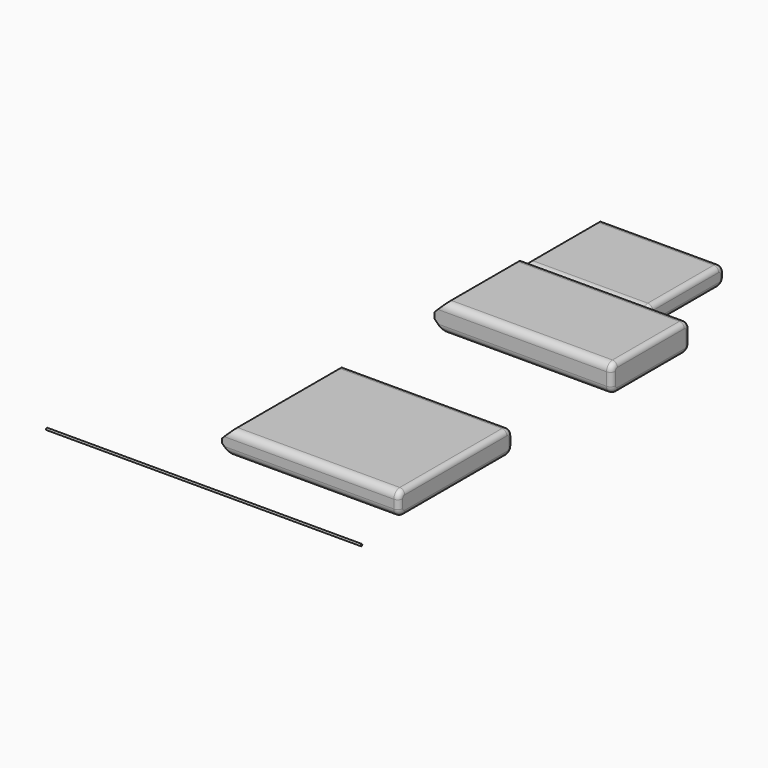
from build123d import *

# Parameters (mm, degrees)
F0_W         = 36
F0_H         = 29
F1_DEPTH     = 4.75
F2_R         = 1.5
F3_T1_DEPTH  = 36.2867319519
F4_R         = 1
F5_W         = 36
F5_H         = 20
F6_DEPTH     = 5.6
F7_R         = 1.5
F8_R         = 1
F9_T1_DEPTH  = 28.3154051471
F10_W        = 26.02
F10_H        = 19.75
F11_DEPTH    = 3.8
F12_R        = 1.5
F13_R        = 1
F14_T1_DEPTH = 24.9793855615
F15_R        = 0.2
F16_DEPTH    = 64


# Not quite as in the source:
# - a fillet or chamfer that OpenCascade refuses, or shapes differently, is made with other operations: its cross-section is extruded or revolved along the edge and cut away or added


with BuildPart() as f1:
    # F0 (on Top) → F1 (new body)
    with BuildSketch(Plane.XY):
        with Locations((18, 14.5)):
            Rectangle(F0_W, F0_H)
    extrude(amount=F1_DEPTH)

    # F2
    f2_edges = [f1.edges().sort_by_distance(p)[0] for p in [
        (18, 0, 4.75),
        (18, 0, 0),
        (18, 29, 4.75),
        (18, 29, 0),
    ]]
    fillet(f2_edges, radius=F2_R)

    # F3: chamfer of 2 on 2 edges, made by hand

    # F3_s2 → F3_t1 (cut)
    with BuildSketch(Plane.XZ.offset(-32.6433659759)):
        Polygon((0, 2), (2, 0), (0, 0), align=None)
        Polygon((0, 2.75), (2, 4.75), (0, 4.75), align=None)
    extrude(amount=F3_T1_DEPTH, mode=Mode.SUBTRACT)

    # F4
    f4_edges = [f1.edges().sort_by_distance(p)[0] for p in [
        (36, 14.5, 4.75),
        (36, 14.5, 0),
    ]]
    fillet(f4_edges, radius=F4_R)


with BuildPart() as f6:
    # F5 (on Top) → F6 (new body)
    with BuildSketch(Plane.XY):
        with Locations((18, 64.0816430916)):
            Rectangle(F5_W, F5_H)
    extrude(amount=F6_DEPTH)

    # F7
    f7_edges = [f6.edges().sort_by_distance(p)[0] for p in [
        (18, 54.081643, 5.6),
        (18, 54.081643, 0),
        (18, 74.081643, 5.6),
        (18, 74.081643, 0),
    ]]
    fillet(f7_edges, radius=F7_R)

    # F8
    f8_edges = [f6.edges().sort_by_distance(p)[0] for p in [
        (36, 64.081643, 5.6),
        (36, 64.081643, 0),
    ]]
    fillet(f8_edges, radius=F8_R)

    # F9: chamfer of 2.2 on 2 edges, made by hand

    # F9_s2 → F9_t1 (cut)
    with BuildSketch(Plane.XZ.offset(-78.2393456652)):
        Polygon((0, 3.4), (2.2, 5.6), (0, 5.6), align=None)
        Polygon((0, 2.2), (2.2, 0), (0, 0), align=None)
    extrude(amount=F9_T1_DEPTH, mode=Mode.SUBTRACT)


with BuildPart() as f11:
    # F10 (on Top) → F11 (new body)
    with BuildSketch(Plane.XY):
        with Locations((13.01, 85.4182140244)):
            Rectangle(F10_W, F10_H)
    extrude(amount=F11_DEPTH)

    # F12
    f12_edges = [f11.edges().sort_by_distance(p)[0] for p in [
        (13.01, 75.543214, 3.8),
        (13.01, 75.543214, 0),
        (13.01, 95.293214, 3.8),
        (13.01, 95.293214, 0),
    ]]
    fillet(f12_edges, radius=F12_R)

    # F13
    f13_edges = [f11.edges().sort_by_distance(p)[0] for p in [
        (26.02, 85.418214, 3.8),
        (26.02, 85.418214, 0),
        (26.02, 95.293214, 1.9),
        (26.02, 94.853874, 0.43934),
        (26.02, 94.853874, 3.36066),
        (26.02, 75.982554, 0.43934),
        (26.02, 75.982554, 3.36066),
        (26.02, 75.543214, 1.9),
    ]]
    fillet(f13_edges, radius=F13_R)

    # F14: chamfer of 1.6 on 2 edges, made by hand

    # F14_s2 → F14_t1 (cut)
    with BuildSketch(Plane.XZ.offset(-97.9079068052)):
        Polygon((0, 2.2), (1.6, 3.8), (0, 3.8), align=None)
        Polygon((0, 1.6), (1.6, 0), (0, 0), align=None)
    extrude(amount=F14_T1_DEPTH, mode=Mode.SUBTRACT)


with BuildPart() as f16:
    # F15 (on Right) → F16 (new body)
    with BuildSketch(Plane.YZ):
        with Locations((-44.4816090167, 22.5465968251)):
            Circle(F15_R)
    extrude(amount=F16_DEPTH)


solid = Compound([f1.part, f6.part, f11.part, f16.part])
